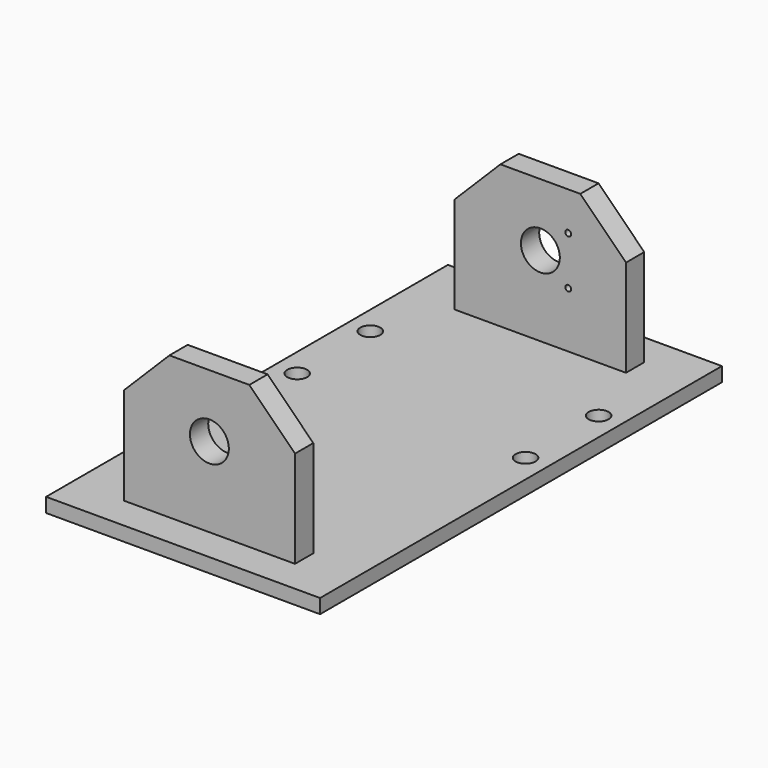
from build123d import *

# Parameters (mm, degrees)
F0_W      = 304.8
F0_H      = 558.8
F1_DEPTH  = 15.875
F3_D      = 22.225
F4_W      = 190.5
F4_H      = 25.4
F5_DEPTH  = 158.75
F6_SIZE   = 50.8
F8_R      = 21.6281
F9_DEPTH  = 522.225
F12_D     = 6.5278
F13_W     = 25.4
F13_H     = 76.2
F13_R     = 3.2639
F14_DEPTH = 6.35


# Not quite as in the source:
# - a length typed as a fraction of an inch, garbled in the dataset ("3 / 203.2 mm" for 3/8 in), is restored


with BuildPart() as f1:
    # F0 (on Top) → F1 (new body)
    with BuildSketch(Plane.XY):
        Rectangle(F0_W, F0_H)
    extrude(amount=-F1_DEPTH)

    # F3 (through all)
    with Locations(Plane.XY):
        with Locations((-127, 139.7), (127, 139.7), (127, 38.1), (-127, 38.1)):
            Hole(F3_D / 2)


with BuildPart() as f5:
    # F4 (on face) → F5 (new body)
    with BuildSketch(Plane.XY):
        with Locations((0, 230.124)):
            Rectangle(F4_W, F4_H)
    extrude(amount=F5_DEPTH)

    # F6
    f6_edges = [f5.edges().sort_by_distance(p)[0] for p in [
        (95.25, 230.124, 158.75),
        (-95.25, 230.124, 158.75),
    ]]
    chamfer(f6_edges, length=F6_SIZE)

    # F8 (on face) → F9 (cut, through all)
    with BuildSketch(Plane(origin=(0, 242.824, 0), x_dir=(-1, 0, 0), z_dir=(0, 1, 0))):
        with Locations((0, 88.9)):
            Circle(F8_R)
    extrude(amount=-F9_DEPTH, mode=Mode.SUBTRACT)


with BuildPart() as f10_1:
    # F10: instance of F5
    add(f5.part.mirror(Plane.XZ))


with BuildPart() as f5_1:
    add(f5.part)

    # F12 (through all)
    with Locations(Plane(origin=(0, 242.824, 0), x_dir=(-1, 0, 0), z_dir=(0, 1, 0))):
        with Locations((-30.988, 115.8748), (-30.988, 61.9252)):
            Hole(F12_D / 2)


with BuildPart() as f14:
    # F13 (on face) → F14 (new body)
    with BuildSketch(Plane(origin=(0, 242.824, 0), x_dir=(-1, 0, 0), z_dir=(0, 1, 0))):
        with Locations((-30.988, 88.9)):
            Rectangle(F13_W, F13_H)
        with Locations((-30.988, 61.9252)):
            Circle(F13_R, mode=Mode.SUBTRACT)
        with Locations((-30.988, 115.8748)):
            Circle(F13_R, mode=Mode.SUBTRACT)
    extrude(amount=F14_DEPTH)


solid = Compound([f1.part, f10_1.part, f5_1.part, f14.part])
